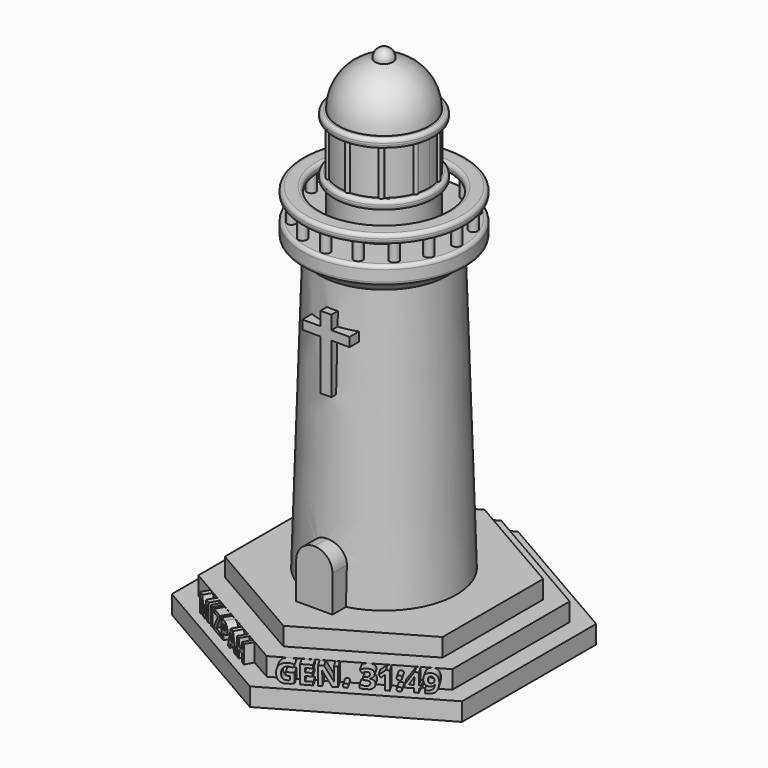
from build123d import *

# Parameters (mm, degrees)
F1_DEPTH      = 3.175
F3_DEPTH      = 3.175
F5_DEPTH      = 3.175
F6_R          = 12.7
F7_DEPTH      = 50.8
F11_DEPTH     = 12.7
F13_R         = 14.2875
F14_DEPTH     = 3.175
F15_R         = 7.9375
F16_DEPTH     = 15.875
F17_R         = 0.79375
F18_DEPTH     = 3.175
F20_R         = 14.2875
F20_R_2       = 11.1125
F21_DEPTH     = 1.5875
F25_R         = 8.89
F25_R_2       = 6.35
F26_DEPTH     = 0.79375
F27_R         = 8.89
F28_DEPTH     = 0.79375
F31_R         = 0.635
F34_W         = 3.175
F34_H         = 6.35
F35_DEPTH     = 15.24
F36_R         = 5.715
F37_DEPTH     = 79.375
F38_R         = 7.9375
F39_DEPTH     = 57.15
F40_TEXT_SIZE = 4.4097222222
F41_DEPTH     = 1.5875
F42_TEXT_SIZE = 4.4097222222
F43_DEPTH     = 1.5875
F45_R         = 0.41275
F46_DEPTH     = 8.89
F47_R         = 6.985
F48_DEPTH     = 7.9375


# Not quite as in the source:
# - Text() gives the source's letters only with a copy of the font that has no kerning and outlines rounded to 1/6400 em; it was checked with that copy


with BuildPart() as f1:
    # F0 (on Top) → F1 (new body)
    with BuildSketch(Plane.XY):
        Polygon((25.4, -14.6646968374), (25.4, 14.6646968374), (0, 29.3293936748), (-25.4, 14.6646968374), (-25.4, -14.6646968374), (0, -29.3293936748), align=None)
    extrude(amount=F1_DEPTH)

    # F2 (on face) → F3 (join)
    with BuildSketch(Plane.XY.offset(3.175)):
        Polygon((22.225, -12.8316097327), (22.225, 12.8316097327), (0, 25.6632194655), (-22.225, 12.8316097327), (-22.225, -12.8316097327), (0, -25.6632194655), align=None)
    extrude(amount=F3_DEPTH)

    # F4 (on face) → F5 (join)
    with BuildSketch(Plane.XY.offset(6.35)):
        Polygon((19.05, -10.9985226281), (19.05, 10.9985226281), (0, 21.9970452561), (-19.05, 10.9985226281), (-19.05, -10.9985226281), (0, -21.9970452561), align=None)
    extrude(amount=F5_DEPTH)

    # F6 (on face) → F7 (join)
    with BuildSketch(Plane.XY.offset(9.525)):
        Circle(F6_R)
    extrude(amount=F7_DEPTH)

    # F8 (on Right) → F9 (revolve, cut)
    with BuildSketch(Plane.YZ):
        Polygon((-12.7, 9.525), (-11.1125, 60.325), (-12.7, 60.325), align=None)
    revolve(axis=Axis((0, 0, 55.6289087981), (0, 0, -1)), mode=Mode.SUBTRACT)

    # F10 (on Front) → F11 (join)
    with BuildSketch(Plane.XZ):
        Polygon((0.9525, 53.975), (0, 53.975), (0, 41.275), (0.9525, 41.275), (0.9525, 50.00625), (4.1275, 50.00625), (4.1275, 51.59375), (0.9525, 51.59375), align=None)
        Polygon((0, 41.275), (0, 53.975), (-0.9525, 53.975), (-0.9525, 51.59375), (-4.1275, 51.59375), (-4.1275, 50.00625), (-0.9525, 50.00625), (-0.9525, 41.275), align=None)
    extrude(amount=F11_DEPTH)

    # F13 (on offset) → F14 (join)
    with BuildSketch(Plane.XY.offset(60.325)):
        Circle(F13_R)
    extrude(amount=F14_DEPTH)

    # F15 (on face) → F16 (join)
    with BuildSketch(Plane.XY.offset(63.5)):
        Circle(F15_R)
    extrude(amount=F16_DEPTH)

    # F17 (on face) → F18 (join)
    with BuildSketch(Plane.XY.offset(63.5)):
        with Locations((0, 12.7)):
            Circle(F17_R)
        with Locations((-4.860079591, 11.7332700629)):
            Circle(F17_R)
        with Locations((-8.9802561211, 8.9802561211)):
            Circle(F17_R)
        with Locations((-11.7332700629, 4.860079591)):
            Circle(F17_R)
        with Locations((-12.7, 0)):
            Circle(F17_R)
        with Locations((-11.7332700629, -4.860079591)):
            Circle(F17_R)
        with Locations((-8.9802561211, -8.9802561211)):
            Circle(F17_R)
        with Locations((-4.860079591, -11.7332700629)):
            Circle(F17_R)
        with Locations((0, -12.7)):
            Circle(F17_R)
        with Locations((4.860079591, -11.7332700629)):
            Circle(F17_R)
        with Locations((8.9802561211, -8.9802561211)):
            Circle(F17_R)
        with Locations((11.7332700629, -4.860079591)):
            Circle(F17_R)
        with Locations((12.7, 0)):
            Circle(F17_R)
        with Locations((11.7332700629, 4.860079591)):
            Circle(F17_R)
        with Locations((8.9802561211, 8.9802561211)):
            Circle(F17_R)
        with Locations((4.860079591, 11.7332700629)):
            Circle(F17_R)
    extrude(amount=F18_DEPTH)

    # F20 (on offset) → F21 (join)
    with BuildSketch(Plane.XY.offset(66.675)):
        Circle(F20_R)
        Circle(F20_R_2, mode=Mode.SUBTRACT)
    extrude(amount=F21_DEPTH)

    # F22 (on Front) → F23 (revolve)
    with BuildSketch(Plane.XZ):
        Polygon((10.795, 60.325), (10.795, 57.785), (13.335, 60.325), align=None)
    revolve(axis=Axis((0, 0, 57.790575549), (0, 0, -1)))

    # F25 (on offset) → F26 (join, symmetric)
    with BuildSketch(Plane.XY.offset(69.85)):
        Circle(F25_R)
        Circle(F25_R_2, mode=Mode.SUBTRACT)
    extrude(amount=F26_DEPTH, both=True)

    # F27 (on face) → F28 (join, symmetric)
    with BuildSketch(Plane.XY.offset(79.375)):
        Circle(F27_R)
    extrude(amount=F28_DEPTH, both=True)

    # F29 (on Front) → F30 (revolve)
    with BuildSketch(Plane.XZ):
        with BuildLine():
            Line((0, 80.16875), (7.9375, 80.16875))
            ThreePointArc((7.9375, 80.16875), (5.6126600757, 85.7814100757), (0, 88.10625))
            Line((0, 88.10625), (0, 80.16875))
        make_face()
    revolve(axis=Axis((0, 0, 84.1375), (0, 0, -1)))

    # F31
    f31_edges = [f1.edges().sort_by_distance(p)[0] for p in [
        (-14.2875, 0, 60.325),
        (-14.2875, 0, 63.5),
        (-8.89, 0, 69.05625),
        (-8.89, 0, 70.64375),
        (-8.89, 0, 78.58125),
        (-8.89, 0, 80.16875),
        (-14.2875, 0, 66.675),
        (-14.2875, 0, 68.2625),
        (-11.1125, 0, 68.2625),
        (-11.1125, 0, 66.675),
    ]]
    fillet(f31_edges, radius=F31_R)

    # F32 (on Front) → F33 (revolve)
    with BuildSketch(Plane.XZ):
        with BuildLine():
            Line((0, 89.69375), (0, 86.51875))
            ThreePointArc((0, 86.51875), (1.5875, 88.10625), (0, 89.69375))
        make_face()
    revolve(axis=Axis((0, 0, 88.10625), (0, 0, -1)))

    # F34 (on Front) → F35 (join)
    with BuildSketch(Plane.XZ):
        with Locations((1.5875, 12.7)):
            Rectangle(F34_W, F34_H)
        with BuildLine():
            Line((-3.175, 9.525), (0, 9.525))
            Line((0, 9.525), (0, 15.875))
            Line((0, 15.875), (3.175, 15.875))
            ThreePointArc((3.175, 15.875), (2.2450640303, 18.1200640303), (0, 19.05))
            ThreePointArc((0, 19.05), (-2.2450640303, 18.1200640303), (-3.175, 15.875))
            Line((-3.175, 15.875), (-3.175, 9.525))
        make_face()
    extrude(amount=F35_DEPTH)

    # F36 (on face) → F37 (cut)
    with BuildSketch(Plane(origin=(0, 0, 0), x_dir=(1, 0, 0), z_dir=(0, 0, -1))):
        Circle(F36_R)
    extrude(amount=-F37_DEPTH, mode=Mode.SUBTRACT)

    # F38 (on face) → F39 (cut)
    with BuildSketch(Plane(origin=(0, 0, 0), x_dir=(1, 0, 0), z_dir=(0, 0, -1))):
        Circle(F38_R)
    extrude(amount=-F39_DEPTH, mode=Mode.SUBTRACT)

    # F40 (on face) → F41 (join)
    with BuildSketch(Plane(origin=(-11.1125, -19.2474145991, 0), x_dir=(0.8660254038, -0.5, 0), z_dir=(-0.5, -0.8660254038, 0))):
        with Locations((-8.6223849826, 3.175)):
            Text('MIZPAH', F40_TEXT_SIZE, font='Open Sans', font_style=FontStyle.BOLD, text_align=(TextAlign.LEFT, TextAlign.BOTTOM))
    extrude(amount=F41_DEPTH)

    # F42 (on face) → F43 (join)
    with BuildSketch(Plane(origin=(11.1125, -19.2474145991, 0), x_dir=(0.8660254038, 0.5, 0), z_dir=(0.5, -0.8660254038, 0))):
        with Locations((-11.5545057509, 3.175)):
            Text('GEN. 31:49', F42_TEXT_SIZE, font='Open Sans', font_style=FontStyle.BOLD, text_align=(TextAlign.LEFT, TextAlign.BOTTOM))
    extrude(amount=F43_DEPTH)

    # F45 (on offset) → F46 (join)
    with BuildSketch(Plane.XY.offset(70.64375)):
        with Locations((0, 7.84225)):
            Circle(F45_R)
        with Locations((-4.6095588948, 6.3445135241)):
            Circle(F45_R)
        with Locations((-7.4584229649, 2.4233885241)):
            Circle(F45_R)
        with Locations((-7.4584229649, -2.4233885241)):
            Circle(F45_R)
        with Locations((-4.6095588948, -6.3445135241)):
            Circle(F45_R)
        with Locations((0, -7.84225)):
            Circle(F45_R)
        with Locations((4.6095588948, -6.3445135241)):
            Circle(F45_R)
        with Locations((7.4584229649, -2.4233885241)):
            Circle(F45_R)
        with Locations((7.4584229649, 2.4233885241)):
            Circle(F45_R)
        with Locations((4.6095588948, 6.3445135241)):
            Circle(F45_R)
    extrude(amount=F46_DEPTH)

    # F47 (on offset) → F48 (cut)
    with BuildSketch(Plane.XY.offset(70.64375)):
        Circle(F47_R)
    extrude(amount=F48_DEPTH, mode=Mode.SUBTRACT)


solid = f1.part
